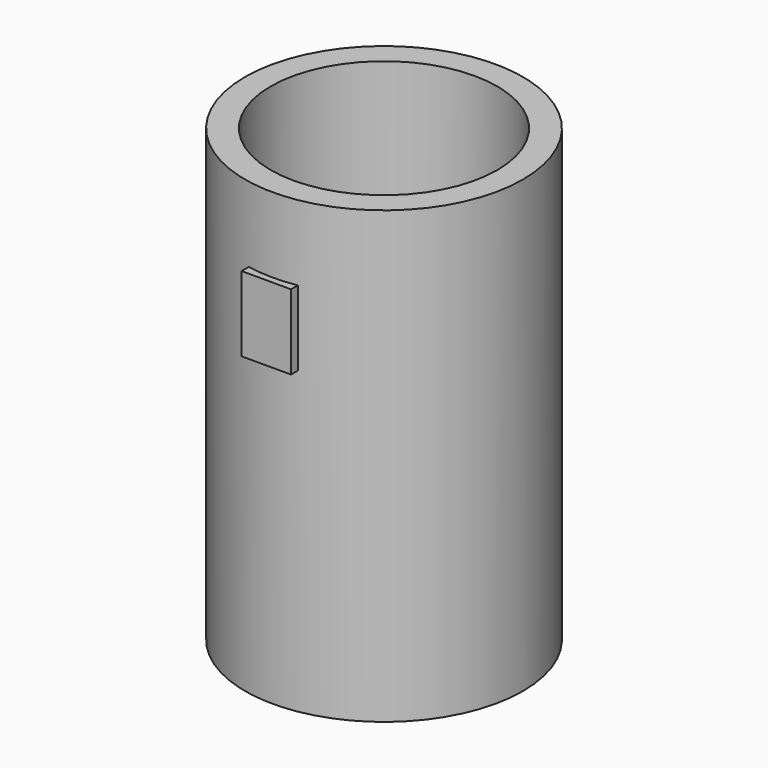
from build123d import *

# Parameters (mm, degrees)
F0_R     = 47.0125269351
F0_R_2   = 38.3432556573
F1_DEPTH = 101.6
F4_DEPTH = 25.4
F5_DEPTH = 25.4
F6_DEPTH = 25.4


with BuildPart() as f1:
    # F0 (on Top) → F1 (new body)
    with BuildSketch(Plane.XY):
        Circle(F0_R)
        Circle(F0_R_2, mode=Mode.SUBTRACT)
    extrude(amount=F1_DEPTH)

    # F4 (add): a face of the model
    f4_faces = [f1.faces().sort_by_distance(p)[0] for p in [
        (-45.6828118712, 0, 101.6),
    ]]
    extrude(f4_faces, amount=F4_DEPTH)

    # F5 (add): a face of the model
    f5_faces = [f1.faces().sort_by_distance(p)[0] for p in [
        (-45.6828118712, 0, 127),
    ]]
    extrude(f5_faces, amount=F5_DEPTH)

    # F3 (on face) → F6 (join)
    with BuildSketch(Plane.XY.offset(101.6)):
        with BuildLine():
            ThreePointArc((7.9259239137, -46.3395880316), (-0.4478621348, -47.0103936202), (-8.8073480874, -46.180172244))
            Line((-8.8073480874, -46.180172244), (-8.8073480874, -49.2319874465))
            Line((-8.8073480874, -49.2319874465), (7.9259239137, -49.2319874465))
            Line((7.9259239137, -49.2319874465), (7.9259239137, -46.3395880316))
        make_face()
    extrude(amount=F6_DEPTH)


solid = f1.part
